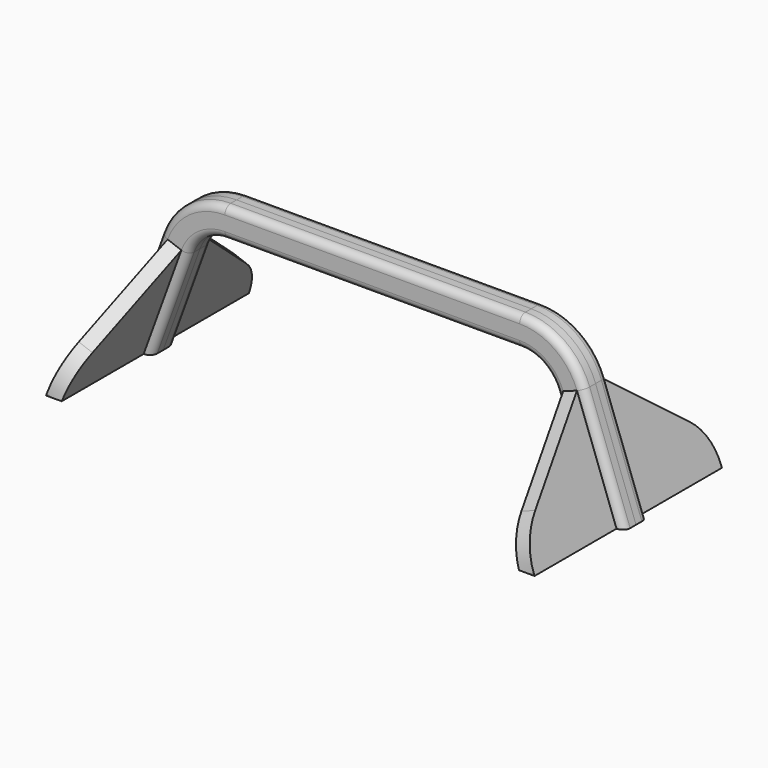
from build123d import *

# Parameters (mm, degrees)
F1_DEPTH = 19.05
F2_DEPTH = 19.05
F3_R     = 9.52499
F3_2_R   = 9.52499
F4_W     = 19.05
F4_H     = 61.2004494442
F5_DEPTH = 19.05
F6_W     = 154.725164175
F6_H     = 323.0141699314
F7_DEPTH = 25.4


# Not quite as in the source:
# - a fillet or chamfer is up to 0.001 mm smaller than in the source, because OpenCascade refuses the exact size


with BuildPart() as f1:
    # F0 (on Front) → F1 (new body)
    with BuildSketch(Plane.XZ):
        with BuildLine():
            Line((191.7515498532, 0), (0, 0))
            Line((0, 0), (-191.7515498532, 0))
            ThreePointArc((-191.7515498532, 0), (-242.7424950448, -16.0773832627), (-275.290223841, -58.4944092583))
            Line((-275.290223841, -58.4944092583), (-327.9587516029, -203.2))
            Line((-327.9587516029, -203.2), (-317.8224583201, -203.2))
            Line((-317.8224583201, -203.2), (-296.8906718296, -145.6903892685))
            Line((-296.8906718296, -145.6903892685), (-278.9895274036, -152.2058729989))
            Line((-278.9895274036, -152.2058729989), (-297.5498717544, -203.2))
            Line((-297.5498717544, -203.2), (-287.4135784716, -203.2))
            Line((-287.4135784716, -203.2), (-239.4879349891, -71.5253767191))
            ThreePointArc((-239.4879349891, -71.5253767191), (-220.8892328198, -47.2870761501), (-191.7515498532, -38.1))
            Line((-191.7515498532, -38.1), (0, -38.1))
            Line((0, -38.1), (191.7515498532, -38.1))
            ThreePointArc((191.7515498532, -38.1), (220.8892328198, -47.2870761501), (239.4879349891, -71.5253767191))
            Line((239.4879349891, -71.5253767191), (287.4135784716, -203.2))
            Line((287.4135784716, -203.2), (297.5498717544, -203.2))
            Line((297.5498717544, -203.2), (278.9895274036, -152.2058729989))
            Line((278.9895274036, -152.2058729989), (296.8906718296, -145.6903892685))
            Line((296.8906718296, -145.6903892685), (317.8224583201, -203.2))
            Line((317.8224583201, -203.2), (327.9587516029, -203.2))
            Line((327.9587516029, -203.2), (275.290223841, -58.4944092583))
            ThreePointArc((275.290223841, -58.4944092583), (242.7424950448, -16.0773832627), (191.7515498532, 0))
        make_face()
    extrude(amount=F1_DEPTH)

    # F3 (radius 9.525 in the source; OpenCascade refuses exactly that, so slightly less here)
    f3_edges = [f1.edges().sort_by_distance(p)[0] for p in [
        (0, -19.05, 0),
        (-242.742495, -19.05, -16.077383),
        (0, -19.05, -38.1),
        (-220.889233, -19.05, -47.287076),
        (220.889233, -19.05, -47.287076),
        (242.742495, -19.05, -16.077383),
    ]]
    fillet(f3_edges, radius=F3_R)


with BuildPart() as f2:
    # F0 (on Front) → F2 (new body)
    with BuildSketch(Plane.XZ):
        with BuildLine():
            Line((191.7515498532, 0), (0, 0))
            Line((0, 0), (-191.7515498532, 0))
            ThreePointArc((-191.7515498532, 0), (-242.7424950448, -16.0773832627), (-275.290223841, -58.4944092583))
            Line((-275.290223841, -58.4944092583), (-327.9587516029, -203.2))
            Line((-327.9587516029, -203.2), (-317.8224583201, -203.2))
            Line((-317.8224583201, -203.2), (-296.8906718296, -145.6903892685))
            Line((-296.8906718296, -145.6903892685), (-278.9895274036, -152.2058729989))
            Line((-278.9895274036, -152.2058729989), (-297.5498717544, -203.2))
            Line((-297.5498717544, -203.2), (-287.4135784716, -203.2))
            Line((-287.4135784716, -203.2), (-239.4879349891, -71.5253767191))
            ThreePointArc((-239.4879349891, -71.5253767191), (-220.8892328198, -47.2870761501), (-191.7515498532, -38.1))
            Line((-191.7515498532, -38.1), (0, -38.1))
            Line((0, -38.1), (191.7515498532, -38.1))
            ThreePointArc((191.7515498532, -38.1), (220.8892328198, -47.2870761501), (239.4879349891, -71.5253767191))
            Line((239.4879349891, -71.5253767191), (287.4135784716, -203.2))
            Line((287.4135784716, -203.2), (297.5498717544, -203.2))
            Line((297.5498717544, -203.2), (278.9895274036, -152.2058729989))
            Line((278.9895274036, -152.2058729989), (296.8906718296, -145.6903892685))
            Line((296.8906718296, -145.6903892685), (317.8224583201, -203.2))
            Line((317.8224583201, -203.2), (327.9587516029, -203.2))
            Line((327.9587516029, -203.2), (275.290223841, -58.4944092583))
            ThreePointArc((275.290223841, -58.4944092583), (242.7424950448, -16.0773832627), (191.7515498532, 0))
        make_face()
    extrude(amount=-F2_DEPTH)

    # F3#2 (radius 9.525 in the source; OpenCascade refuses exactly that, so slightly less here)
    f3_2_edges = [f2.edges().sort_by_distance(p)[0] for p in [
        (-242.742495, 19.05, -16.077383),
        (0, 19.05, 0),
        (242.742495, 19.05, -16.077383),
        (220.889233, 19.05, -47.287076),
        (0, 19.05, -38.1),
    ]]
    fillet(f3_2_edges, radius=F3_2_R)


with BuildPart() as f5:
    # F4 (on face) → F5 (new body)
    with BuildSketch(Plane(origin=(-215.3370720631, 0, 78.376284565), x_dir=(0, 1, 0), z_dir=(0.9396926208, 0, -0.3420201433))):
        with Locations((9.525, -269.0469985684)):
            Rectangle(F4_W, F4_H)
        with Locations((-9.525, -269.0469985684)):
            Rectangle(F4_W, F4_H)
        with BuildLine():
            Line((-152.4, -296.9716030201), (-152.4, -299.6472232904))
            Line((-152.4, -299.6472232904), (-19.05, -299.6472232904))
            Line((-19.05, -299.6472232904), (-19.05, -238.4467738463))
            Line((-19.05, -238.4467738463), (-19.05, -149.1215665516))
            Line((-19.05, -149.1215665516), (-125.3166007179, -238.7135603657))
            ThreePointArc((-125.3166007179, -238.7135603657), (-145.2982090025, -264.8487527006), (-152.4, -296.9716030201))
        make_face()
        with BuildLine():
            Line((19.05, -238.4467738463), (19.05, -299.6472232904))
            Line((19.05, -299.6472232904), (152.4, -299.6472232904))
            Line((152.4, -299.6472232904), (152.4, -296.9716030201))
            ThreePointArc((152.4, -296.9716030201), (145.2982090025, -264.8487527006), (125.3166007179, -238.7135603657))
            Line((125.3166007179, -238.7135603657), (19.05, -149.1215665516))
            Line((19.05, -149.1215665516), (19.05, -238.4467738463))
        make_face()
    extrude(amount=F5_DEPTH)

    # F6 (on face) → F7 (cut)
    with BuildSketch(Plane(origin=(0, 0, -203.2), x_dir=(1, 0, 0), z_dir=(0, 0, -1))):
        with Locations((-313.482388854, -5.5776387453)):
            Rectangle(F6_W, F6_H)
    extrude(amount=F7_DEPTH, mode=Mode.SUBTRACT)


with BuildPart() as f8_1:
    # F8: instance of F5
    add(f5.part.mirror(Plane.YZ))


solid = Compound([f1.part, f2.part, f5.part, f8_1.part])
